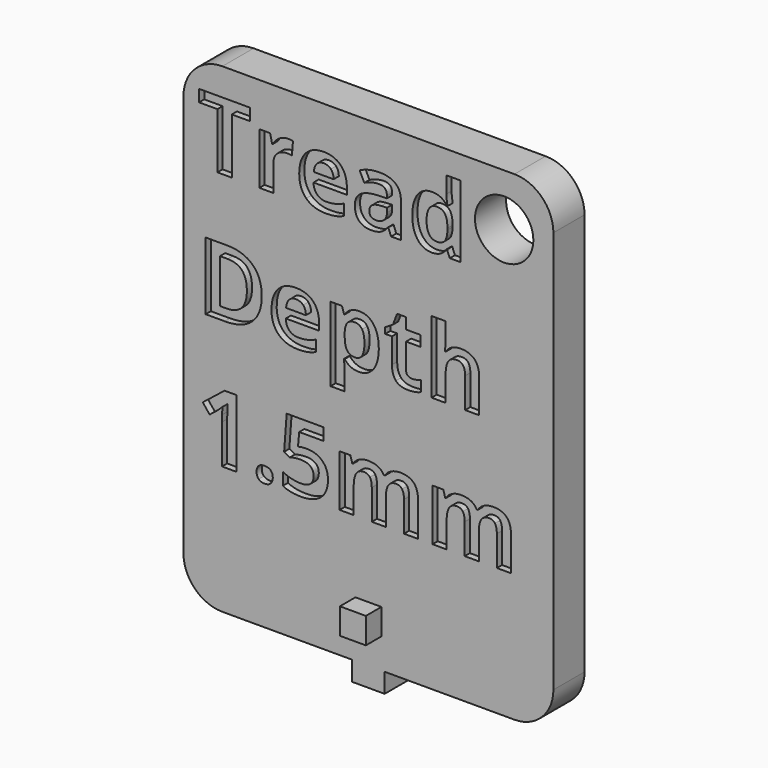
from build123d import *

# Parameters (mm, degrees)
F0_W         = 2
F0_H         = 2
F0_R         = 2.25
F1_DEPTH     = 3
F0_TEXT_SIZE = 7.2916666667
F2_DEPTH     = 2.5
F3_DEPTH     = 4.5
F4_R         = 3


# Not quite as in the source:
# - Text() gives the source's letters only with a copy of the font that has no kerning and outlines rounded to 1/6400 em; it was checked with that copy


with BuildPart() as f1:
    # F0 (on Front) → F1 (new body)
    with BuildSketch(Plane.XZ):
        Polygon((-22.369877694, 72.3569517974), (-50.869877694, 72.3569517974), (-50.869877694, 35.3569517974), (-37.869877694, 35.3569517974), (-37.869877694, 33.8569517974), (-35.369877694, 33.8569517974), (-35.369877694, 35.3569517974), (-22.369877694, 35.3569517974), align=None)
        with BuildLine():
            Line((-46.8008372088, 50.4102206628), (-46.8008372088, 45.2046542565))
            Line((-46.8008372088, 45.2046542565), (-47.9014231463, 45.2046542565))
            Line((-47.9014231463, 45.2046542565), (-47.9014231463, 48.2170240482))
            Line((-47.9014231463, 48.2170240482), (-47.8900299172, 48.711490194))
            Line((-47.8900299172, 48.711490194), (-47.8729400734, 49.2526685794))
            add(Edge.make_bspline(
                [(-47.8729400734, 49.2526685794), (-48.1463775734, 48.9792310794), (-48.2534739276, 48.8937818607)],
                knots=[0, 0, 0, 1, 1, 1], degree=2))
            Line((-48.2534739276, 48.8937818607), (-48.8516184588, 48.4129875898))
            Line((-48.8516184588, 48.4129875898), (-49.382542938, 49.0749342044))
            Line((-49.382542938, 49.0749342044), (-47.7054596047, 50.4102206628))
            Line((-47.7054596047, 50.4102206628), (-46.8008372088, 50.4102206628))
        make_face(mode=Mode.SUBTRACT)
        with BuildLine():
            add(Edge.make_bspline(
                [(-45.0707753599, 45.2673170169), (-45.2342681984, 45.4256829023), (-45.2342681984, 45.7139316003)],
                knots=[0, 0, 0, 1, 1, 1], degree=2))
            add(Edge.make_bspline(
                [(-45.2342681984, 45.7139316003), (-45.2342681984, 46.0124342044), (-45.0741933286, 46.1656731367)],
                knots=[0, 0, 0, 1, 1, 1], degree=2))
            add(Edge.make_bspline(
                [(-45.0741933286, 46.1656731367), (-44.9141184588, 46.318912069), (-44.6076405942, 46.318912069)],
                knots=[0, 0, 0, 1, 1, 1], degree=2))
            add(Edge.make_bspline(
                [(-44.6076405942, 46.318912069), (-44.3125559588, 46.318912069), (-44.1507721047, 46.162255168)],
                knots=[0, 0, 0, 1, 1, 1], degree=2))
            add(Edge.make_bspline(
                [(-44.1507721047, 46.162255168), (-43.9889882505, 46.0055982669), (-43.9889882505, 45.7139316003)],
                knots=[0, 0, 0, 1, 1, 1], degree=2))
            add(Edge.make_bspline(
                [(-43.9889882505, 45.7139316003), (-43.9889882505, 45.4325188398), (-44.152481089, 45.2707349857)],
                knots=[0, 0, 0, 1, 1, 1], degree=2))
            add(Edge.make_bspline(
                [(-44.152481089, 45.2707349857), (-44.3159739276, 45.1089511315), (-44.6076405942, 45.1089511315)],
                knots=[0, 0, 0, 1, 1, 1], degree=2))
            add(Edge.make_bspline(
                [(-44.6076405942, 45.1089511315), (-44.9072825213, 45.1089511315), (-45.0707753599, 45.2673170169)],
                knots=[0, 0, 0, 1, 1, 1], degree=2))
        make_face(mode=Mode.SUBTRACT)
        with BuildLine():
            add(Edge.make_bspline(
                [(-41.9233958026, 48.4802076419), (-41.7057851255, 48.5303378503), (-41.3856353859, 48.5303378503)],
                knots=[0, 0, 0, 1, 1, 1], degree=2))
            add(Edge.make_bspline(
                [(-41.3856353859, 48.5303378503), (-40.6314036151, 48.5303378503), (-40.1842193703, 48.1065097253)],
                knots=[0, 0, 0, 1, 1, 1], degree=2))
            add(Edge.make_bspline(
                [(-40.1842193703, 48.1065097253), (-39.7370351255, 47.6826816003), (-39.7370351255, 46.9455396732)],
                knots=[0, 0, 0, 1, 1, 1], degree=2))
            add(Edge.make_bspline(
                [(-39.7370351255, 46.9455396732), (-39.7370351255, 46.0739576419), (-40.2747955422, 45.6034172773)],
                knots=[0, 0, 0, 1, 1, 1], degree=2))
            add(Edge.make_bspline(
                [(-40.2747955422, 45.6034172773), (-40.8125559588, 45.1328769128), (-41.8128814797, 45.1328769128)],
                knots=[0, 0, 0, 1, 1, 1], degree=2))
            add(Edge.make_bspline(
                [(-41.8128814797, 45.1328769128), (-42.6821848651, 45.1328769128), (-43.2153879901, 45.4142896732)],
                knots=[0, 0, 0, 1, 1, 1], degree=2))
            Line((-43.2153879901, 45.4142896732), (-43.2153879901, 46.3656243086))
            add(Edge.make_bspline(
                [(-43.2153879901, 46.3656243086), (-42.9351145526, 46.2163730065), (-42.5608469745, 46.1218092044)],
                knots=[0, 0, 0, 1, 1, 1], degree=2))
            add(Edge.make_bspline(
                [(-42.5608469745, 46.1218092044), (-42.1865793963, 46.0272454023), (-41.8527577817, 46.0272454023)],
                knots=[0, 0, 0, 1, 1, 1], degree=2))
            add(Edge.make_bspline(
                [(-41.8527577817, 46.0272454023), (-40.8444570005, 46.0272454023), (-40.8444570005, 46.8532545169)],
                knots=[0, 0, 0, 1, 1, 1], degree=2))
            add(Edge.make_bspline(
                [(-40.8444570005, 46.8532545169), (-40.8444570005, 47.6405266523), (-41.8880767922, 47.6405266523)],
                knots=[0, 0, 0, 1, 1, 1], degree=2))
            add(Edge.make_bspline(
                [(-41.8880767922, 47.6405266523), (-42.0760650734, 47.6405266523), (-42.3039296567, 47.6029289961)],
                knots=[0, 0, 0, 1, 1, 1], degree=2))
            add(Edge.make_bspline(
                [(-42.3039296567, 47.6029289961), (-42.5317942401, 47.5653313398), (-42.6742096047, 47.522037069)],
                knots=[0, 0, 0, 1, 1, 1], degree=2))
            Line((-42.6742096047, 47.522037069), (-43.1128489276, 47.7578769128))
            Line((-43.1128489276, 47.7578769128), (-42.9168853859, 50.4102206628))
            Line((-42.9168853859, 50.4102206628), (-40.0936431984, 50.4102206628))
            Line((-40.0936431984, 50.4102206628), (-40.0936431984, 49.477115194))
            Line((-40.0936431984, 49.477115194), (-41.9518788755, 49.477115194))
            Line((-41.9518788755, 49.477115194), (-42.0475820005, 48.4551425378))
            Line((-42.0475820005, 48.4551425378), (-41.9233958026, 48.4802076419))
        make_face(mode=Mode.SUBTRACT)
        with Locations((-36.619877694, 38.6735366881)):
            Rectangle(F0_W, F0_H, mode=Mode.SUBTRACT)
        with BuildLine():
            Line((-35.2765859067, 47.2018873294), (-35.2765859067, 45.2046542565))
            Line((-35.2765859067, 45.2046542565), (-36.3623606463, 45.2046542565))
            Line((-36.3623606463, 45.2046542565), (-36.3623606463, 47.5300123294))
            add(Edge.make_bspline(
                [(-36.3623606463, 47.5300123294), (-36.3623606463, 47.9606763919), (-36.5064849953, 48.1760084232)],
                knots=[0, 0, 0, 1, 1, 1], degree=2))
            add(Edge.make_bspline(
                [(-36.5064849953, 48.1760084232), (-36.6506093442, 48.3913404544), (-36.9605051776, 48.3913404544)],
                knots=[0, 0, 0, 1, 1, 1], degree=2))
            add(Edge.make_bspline(
                [(-36.9605051776, 48.3913404544), (-37.3774973651, 48.3913404544), (-37.5660553078, 48.0848625898)],
                knots=[0, 0, 0, 1, 1, 1], degree=2))
            add(Edge.make_bspline(
                [(-37.5660553078, 48.0848625898), (-37.7546132505, 47.7783847253), (-37.7546132505, 47.0777011315)],
                knots=[0, 0, 0, 1, 1, 1], degree=2))
            Line((-37.7546132505, 47.0777011315), (-37.7546132505, 45.2046542565))
            Line((-37.7546132505, 45.2046542565), (-38.8403879901, 45.2046542565))
            Line((-38.8403879901, 45.2046542565), (-38.8403879901, 49.1854485273))
            Line((-38.8403879901, 49.1854485273), (-38.0109609067, 49.1854485273))
            Line((-38.0109609067, 49.1854485273), (-37.8651275734, 48.6761711836))
            Line((-37.8651275734, 48.6761711836), (-37.8047434588, 48.6761711836))
            add(Edge.make_bspline(
                [(-37.8047434588, 48.6761711836), (-37.6440989276, 48.9507480065), (-37.3416086932, 49.1051262617)],
                knots=[0, 0, 0, 1, 1, 1], degree=2))
            add(Edge.make_bspline(
                [(-37.3416086932, 49.1051262617), (-37.0391184588, 49.2595045169), (-36.6471913755, 49.2595045169)],
                knots=[0, 0, 0, 1, 1, 1], degree=2))
            add(Edge.make_bspline(
                [(-36.6471913755, 49.2595045169), (-35.7539622088, 49.2595045169), (-35.4360911151, 48.6761711836)],
                knots=[0, 0, 0, 1, 1, 1], degree=2))
            Line((-35.4360911151, 48.6761711836), (-35.3403879901, 48.6761711836))
            add(Edge.make_bspline(
                [(-35.3403879901, 48.6761711836), (-35.1797434588, 48.9541659753), (-34.8687083026, 49.1068352461)],
                knots=[0, 0, 0, 1, 1, 1], degree=2))
            add(Edge.make_bspline(
                [(-34.8687083026, 49.1068352461), (-34.5576731463, 49.2595045169), (-34.165746063, 49.2595045169)],
                knots=[0, 0, 0, 1, 1, 1], degree=2))
            add(Edge.make_bspline(
                [(-34.165746063, 49.2595045169), (-33.4889882505, 49.2595045169), (-33.1420644224, 48.9125806888)],
                knots=[0, 0, 0, 1, 1, 1], degree=2))
            add(Edge.make_bspline(
                [(-33.1420644224, 48.9125806888), (-32.7951405942, 48.5656568607), (-32.7951405942, 47.8000318607)],
                knots=[0, 0, 0, 1, 1, 1], degree=2))
            Line((-32.7951405942, 47.8000318607), (-32.7951405942, 45.2046542565))
            Line((-32.7951405942, 45.2046542565), (-33.8843333026, 45.2046542565))
            Line((-33.8843333026, 45.2046542565), (-33.8843333026, 47.5300123294))
            add(Edge.make_bspline(
                [(-33.8843333026, 47.5300123294), (-33.8843333026, 47.9606763919), (-34.0284576515, 48.1760084232)],
                knots=[0, 0, 0, 1, 1, 1], degree=2))
            add(Edge.make_bspline(
                [(-34.0284576515, 48.1760084232), (-34.1725820005, 48.3913404544), (-34.4824778338, 48.3913404544)],
                knots=[0, 0, 0, 1, 1, 1], degree=2))
            add(Edge.make_bspline(
                [(-34.4824778338, 48.3913404544), (-34.8812408547, 48.3913404544), (-35.0789133807, 48.1065097253)],
                knots=[0, 0, 0, 1, 1, 1], degree=2))
            add(Edge.make_bspline(
                [(-35.0789133807, 48.1065097253), (-35.2765859067, 47.8216789961), (-35.2765859067, 47.2018873294)],
                knots=[0, 0, 0, 1, 1, 1], degree=2))
        make_face(mode=Mode.SUBTRACT)
        with BuildLine():
            Line((-28.1170806984, 47.2018873294), (-28.1170806984, 45.2046542565))
            Line((-28.1170806984, 45.2046542565), (-29.202855438, 45.2046542565))
            Line((-29.202855438, 45.2046542565), (-29.202855438, 47.5300123294))
            add(Edge.make_bspline(
                [(-29.202855438, 47.5300123294), (-29.202855438, 47.9606763919), (-29.346979787, 48.1760084232)],
                knots=[0, 0, 0, 1, 1, 1], degree=2))
            add(Edge.make_bspline(
                [(-29.346979787, 48.1760084232), (-29.4911041359, 48.3913404544), (-29.8009999692, 48.3913404544)],
                knots=[0, 0, 0, 1, 1, 1], degree=2))
            add(Edge.make_bspline(
                [(-29.8009999692, 48.3913404544), (-30.2179921567, 48.3913404544), (-30.4065500995, 48.0848625898)],
                knots=[0, 0, 0, 1, 1, 1], degree=2))
            add(Edge.make_bspline(
                [(-30.4065500995, 48.0848625898), (-30.5951080422, 47.7783847253), (-30.5951080422, 47.0777011315)],
                knots=[0, 0, 0, 1, 1, 1], degree=2))
            Line((-30.5951080422, 47.0777011315), (-30.5951080422, 45.2046542565))
            Line((-30.5951080422, 45.2046542565), (-31.6808827817, 45.2046542565))
            Line((-31.6808827817, 45.2046542565), (-31.6808827817, 49.1854485273))
            Line((-31.6808827817, 49.1854485273), (-30.8514556984, 49.1854485273))
            Line((-30.8514556984, 49.1854485273), (-30.7056223651, 48.6761711836))
            Line((-30.7056223651, 48.6761711836), (-30.6452382505, 48.6761711836))
            add(Edge.make_bspline(
                [(-30.6452382505, 48.6761711836), (-30.4845937192, 48.9507480065), (-30.1821034849, 49.1051262617)],
                knots=[0, 0, 0, 1, 1, 1], degree=2))
            add(Edge.make_bspline(
                [(-30.1821034849, 49.1051262617), (-29.8796132505, 49.2595045169), (-29.4876861672, 49.2595045169)],
                knots=[0, 0, 0, 1, 1, 1], degree=2))
            add(Edge.make_bspline(
                [(-29.4876861672, 49.2595045169), (-28.5944570005, 49.2595045169), (-28.2765859067, 48.6761711836)],
                knots=[0, 0, 0, 1, 1, 1], degree=2))
            Line((-28.2765859067, 48.6761711836), (-28.1808827817, 48.6761711836))
            add(Edge.make_bspline(
                [(-28.1808827817, 48.6761711836), (-28.0202382505, 48.9541659753), (-27.7092030942, 49.1068352461)],
                knots=[0, 0, 0, 1, 1, 1], degree=2))
            add(Edge.make_bspline(
                [(-27.7092030942, 49.1068352461), (-27.398167938, 49.2595045169), (-27.0062408547, 49.2595045169)],
                knots=[0, 0, 0, 1, 1, 1], degree=2))
            add(Edge.make_bspline(
                [(-27.0062408547, 49.2595045169), (-26.3294830422, 49.2595045169), (-25.982559214, 48.9125806888)],
                knots=[0, 0, 0, 1, 1, 1], degree=2))
            add(Edge.make_bspline(
                [(-25.982559214, 48.9125806888), (-25.6356353859, 48.5656568607), (-25.6356353859, 47.8000318607)],
                knots=[0, 0, 0, 1, 1, 1], degree=2))
            Line((-25.6356353859, 47.8000318607), (-25.6356353859, 45.2046542565))
            Line((-25.6356353859, 45.2046542565), (-26.7248280942, 45.2046542565))
            Line((-26.7248280942, 45.2046542565), (-26.7248280942, 47.5300123294))
            add(Edge.make_bspline(
                [(-26.7248280942, 47.5300123294), (-26.7248280942, 47.9606763919), (-26.8689524432, 48.1760084232)],
                knots=[0, 0, 0, 1, 1, 1], degree=2))
            add(Edge.make_bspline(
                [(-26.8689524432, 48.1760084232), (-27.0130767922, 48.3913404544), (-27.3229726255, 48.3913404544)],
                knots=[0, 0, 0, 1, 1, 1], degree=2))
            add(Edge.make_bspline(
                [(-27.3229726255, 48.3913404544), (-27.7217356463, 48.3913404544), (-27.9194081724, 48.1065097253)],
                knots=[0, 0, 0, 1, 1, 1], degree=2))
            add(Edge.make_bspline(
                [(-27.9194081724, 48.1065097253), (-28.1170806984, 47.8216789961), (-28.1170806984, 47.2018873294)],
                knots=[0, 0, 0, 1, 1, 1], degree=2))
        make_face(mode=Mode.SUBTRACT)
        with BuildLine():
            add(Edge.make_bspline(
                [(-45.5441640317, 59.6541171471), (-44.8389231463, 58.9813469648), (-44.8389231463, 57.7736646732)],
                knots=[0, 0, 0, 1, 1, 1], degree=2))
            add(Edge.make_bspline(
                [(-44.8389231463, 57.7736646732), (-44.8389231463, 56.4885084232), (-45.5709381203, 55.8049146732)],
                knots=[0, 0, 0, 1, 1, 1], degree=2))
            add(Edge.make_bspline(
                [(-45.5709381203, 55.8049146732), (-46.3029530942, 55.1213209232), (-47.6838124692, 55.1213209232)],
                knots=[0, 0, 0, 1, 1, 1], degree=2))
            Line((-47.6838124692, 55.1213209232), (-49.1580963234, 55.1213209232))
            Line((-49.1580963234, 55.1213209232), (-49.1580963234, 60.3268873294))
            Line((-49.1580963234, 60.3268873294), (-47.5243072609, 60.3268873294))
            add(Edge.make_bspline(
                [(-47.5243072609, 60.3268873294), (-46.2494049172, 60.3268873294), (-45.5441640317, 59.6541171471)],
                knots=[0, 0, 0, 1, 1, 1], degree=2))
        make_face(mode=Mode.SUBTRACT)
        with BuildLine():
            add(Edge.make_bspline(
                [(-41.2534739276, 55.1190422773), (-41.5770416359, 55.0495435794), (-42.0441640317, 55.0495435794)],
                knots=[0, 0, 0, 1, 1, 1], degree=2))
            add(Edge.make_bspline(
                [(-42.0441640317, 55.0495435794), (-43.0046132505, 55.0495435794), (-43.5457916359, 55.5804680586)],
                knots=[0, 0, 0, 1, 1, 1], degree=2))
            add(Edge.make_bspline(
                [(-43.5457916359, 55.5804680586), (-44.0869700213, 56.1113925378), (-44.0869700213, 57.0832349857)],
                knots=[0, 0, 0, 1, 1, 1], degree=2))
            add(Edge.make_bspline(
                [(-44.0869700213, 57.0832349857), (-44.0869700213, 58.0835605065), (-43.5868072609, 58.629865845)],
                knots=[0, 0, 0, 1, 1, 1], degree=2))
            add(Edge.make_bspline(
                [(-43.5868072609, 58.629865845), (-43.0866445005, 59.1761711836), (-42.2036692401, 59.1761711836)],
                knots=[0, 0, 0, 1, 1, 1], degree=2))
            add(Edge.make_bspline(
                [(-42.2036692401, 59.1761711836), (-41.3605702817, 59.1761711836), (-40.8905995786, 58.6959465742)],
                knots=[0, 0, 0, 1, 1, 1], degree=2))
            add(Edge.make_bspline(
                [(-40.8905995786, 58.6959465742), (-40.4206288755, 58.2157219648), (-40.4206288755, 57.3680657148)],
                knots=[0, 0, 0, 1, 1, 1], degree=2))
            Line((-40.4206288755, 57.3680657148), (-40.4206288755, 56.8405592044))
            Line((-40.4206288755, 56.8405592044), (-42.9875234067, 56.8405592044))
            add(Edge.make_bspline(
                [(-42.9875234067, 56.8405592044), (-42.9692942401, 56.3779941003), (-42.7129465838, 56.1182284753)],
                knots=[0, 0, 0, 1, 1, 1], degree=2))
            add(Edge.make_bspline(
                [(-42.7129465838, 56.1182284753), (-42.4565989276, 55.8584628503), (-41.9940338234, 55.8584628503)],
                knots=[0, 0, 0, 1, 1, 1], degree=2))
            add(Edge.make_bspline(
                [(-41.9940338234, 55.8584628503), (-41.6340077817, 55.8584628503), (-41.3138580422, 55.9330885013)],
                knots=[0, 0, 0, 1, 1, 1], degree=2))
            add(Edge.make_bspline(
                [(-41.3138580422, 55.9330885013), (-40.9937083026, 56.0077141523), (-40.6450754901, 56.1717766523)],
                knots=[0, 0, 0, 1, 1, 1], degree=2))
            Line((-40.6450754901, 56.1717766523), (-40.6450754901, 55.3309563398))
            add(Edge.make_bspline(
                [(-40.6450754901, 55.3309563398), (-40.9299062192, 55.1885409753), (-41.2534739276, 55.1190422773)],
                knots=[0, 0, 0, 1, 1, 1], degree=2))
        make_face(mode=Mode.SUBTRACT)
        with BuildLine():
            add(Edge.make_bspline(
                [(-36.5400950213, 55.2956373294), (-36.8853098651, 55.0495435794), (-37.351292938, 55.0495435794)],
                knots=[0, 0, 0, 1, 1, 1], degree=2))
            add(Edge.make_bspline(
                [(-37.351292938, 55.0495435794), (-38.0531158547, 55.0495435794), (-38.4518788755, 55.5588209232)],
                knots=[0, 0, 0, 1, 1, 1], degree=2))
            Line((-38.4518788755, 55.5588209232), (-38.5088450213, 55.5588209232))
            add(Edge.make_bspline(
                [(-38.5088450213, 55.5588209232), (-38.4518788755, 55.0609368086), (-38.4518788755, 54.9823235273)],
                knots=[0, 0, 0, 1, 1, 1], degree=2))
            Line((-38.4518788755, 54.9823235273), (-38.4518788755, 53.3690422773))
            Line((-38.4518788755, 53.3690422773), (-39.5376536151, 53.3690422773))
            Line((-39.5376536151, 53.3690422773), (-39.5376536151, 59.102115194))
            Line((-39.5376536151, 59.102115194), (-38.6546783547, 59.102115194))
            Line((-38.6546783547, 59.102115194), (-38.5020090838, 58.5860019128))
            Line((-38.5020090838, 58.5860019128), (-38.4518788755, 58.5860019128))
            add(Edge.make_bspline(
                [(-38.4518788755, 58.5860019128), (-38.0702056984, 59.1761711836), (-37.3228098651, 59.1761711836)],
                knots=[0, 0, 0, 1, 1, 1], degree=2))
            add(Edge.make_bspline(
                [(-37.3228098651, 59.1761711836), (-36.6175689797, 59.1761711836), (-36.2188059588, 58.6315748294)],
                knots=[0, 0, 0, 1, 1, 1], degree=2))
            add(Edge.make_bspline(
                [(-36.2188059588, 58.6315748294), (-35.820042938, 58.0869784753), (-35.820042938, 57.1185539961)],
                knots=[0, 0, 0, 1, 1, 1], degree=2))
            add(Edge.make_bspline(
                [(-35.820042938, 57.1185539961), (-35.820042938, 56.4816724857), (-36.0074615578, 56.0117017825)],
                knots=[0, 0, 0, 1, 1, 1], degree=2))
            add(Edge.make_bspline(
                [(-36.0074615578, 56.0117017825), (-36.1948801776, 55.5417310794), (-36.5400950213, 55.2956373294)],
                knots=[0, 0, 0, 1, 1, 1], degree=2))
        make_face(mode=Mode.SUBTRACT)
        Polygon((-47.1494700213, 69.3252597253), (-47.1494700213, 65.0379875898), (-48.2534739276, 65.0379875898), (-48.2534739276, 69.3252597253), (-49.6673736672, 69.3252597253), (-49.6673736672, 70.2435539961), (-45.7367096047, 70.2435539961), (-45.7367096047, 69.3252597253), align=None, mode=Mode.SUBTRACT)
        with BuildLine():
            add(Edge.make_bspline(
                [(-43.4848378599, 68.8883293867), (-43.1698150734, 69.0928378503), (-42.7995351255, 69.0928378503)],
                knots=[0, 0, 0, 1, 1, 1], degree=2))
            add(Edge.make_bspline(
                [(-42.7995351255, 69.0928378503), (-42.5785064797, 69.0928378503), (-42.4326731463, 69.0609368086)],
                knots=[0, 0, 0, 1, 1, 1], degree=2))
            Line((-42.4326731463, 69.0609368086), (-42.5147043963, 68.043521444))
            add(Edge.make_bspline(
                [(-42.5147043963, 68.043521444), (-42.6468658547, 68.0788404544), (-42.8348541359, 68.0788404544)],
                knots=[0, 0, 0, 1, 1, 1], degree=2))
            add(Edge.make_bspline(
                [(-42.8348541359, 68.0788404544), (-43.3543853859, 68.0788404544), (-43.6449127297, 67.8116692305)],
                knots=[0, 0, 0, 1, 1, 1], degree=2))
            add(Edge.make_bspline(
                [(-43.6449127297, 67.8116692305), (-43.9354400734, 67.5444980065), (-43.9354400734, 67.0637037357)],
                knots=[0, 0, 0, 1, 1, 1], degree=2))
            Line((-43.9354400734, 67.0637037357), (-43.9354400734, 65.0379875898))
            Line((-43.9354400734, 65.0379875898), (-45.021214813, 65.0379875898))
            Line((-45.021214813, 65.0379875898), (-45.021214813, 69.0187818607))
            Line((-45.021214813, 69.0187818607), (-44.1986236672, 69.0187818607))
            Line((-44.1986236672, 69.0187818607), (-44.0379791359, 68.3488599857))
            Line((-44.0379791359, 68.3488599857), (-43.9855702817, 68.3488599857))
            add(Edge.make_bspline(
                [(-43.9855702817, 68.3488599857), (-43.7998606463, 68.6838209232), (-43.4848378599, 68.8883293867)],
                knots=[0, 0, 0, 1, 1, 1], degree=2))
        make_face(mode=Mode.SUBTRACT)
        with BuildLine():
            add(Edge.make_bspline(
                [(-39.1183827817, 65.035708944), (-39.4419504901, 64.9662102461), (-39.9090728859, 64.9662102461)],
                knots=[0, 0, 0, 1, 1, 1], degree=2))
            add(Edge.make_bspline(
                [(-39.9090728859, 64.9662102461), (-40.8695221047, 64.9662102461), (-41.4107004901, 65.4971347253)],
                knots=[0, 0, 0, 1, 1, 1], degree=2))
            add(Edge.make_bspline(
                [(-41.4107004901, 65.4971347253), (-41.9518788755, 66.0280592044), (-41.9518788755, 66.9999016523)],
                knots=[0, 0, 0, 1, 1, 1], degree=2))
            add(Edge.make_bspline(
                [(-41.9518788755, 66.9999016523), (-41.9518788755, 68.0002271732), (-41.4517161151, 68.5465325117)],
                knots=[0, 0, 0, 1, 1, 1], degree=2))
            add(Edge.make_bspline(
                [(-41.4517161151, 68.5465325117), (-40.9515533547, 69.0928378503), (-40.0685780942, 69.0928378503)],
                knots=[0, 0, 0, 1, 1, 1], degree=2))
            add(Edge.make_bspline(
                [(-40.0685780942, 69.0928378503), (-39.2254791359, 69.0928378503), (-38.7555084328, 68.6126132409)],
                knots=[0, 0, 0, 1, 1, 1], degree=2))
            add(Edge.make_bspline(
                [(-38.7555084328, 68.6126132409), (-38.2855377297, 68.1323886315), (-38.2855377297, 67.2847323815)],
                knots=[0, 0, 0, 1, 1, 1], degree=2))
            Line((-38.2855377297, 67.2847323815), (-38.2855377297, 66.7572258711))
            Line((-38.2855377297, 66.7572258711), (-40.8524322609, 66.7572258711))
            add(Edge.make_bspline(
                [(-40.8524322609, 66.7572258711), (-40.8342030942, 66.2946607669), (-40.577855438, 66.0348951419)],
                knots=[0, 0, 0, 1, 1, 1], degree=2))
            add(Edge.make_bspline(
                [(-40.577855438, 66.0348951419), (-40.3215077817, 65.7751295169), (-39.8589426776, 65.7751295169)],
                knots=[0, 0, 0, 1, 1, 1], degree=2))
            add(Edge.make_bspline(
                [(-39.8589426776, 65.7751295169), (-39.4989166359, 65.7751295169), (-39.1787668963, 65.849755168)],
                knots=[0, 0, 0, 1, 1, 1], degree=2))
            add(Edge.make_bspline(
                [(-39.1787668963, 65.849755168), (-38.8586171567, 65.924380819), (-38.5099843442, 66.088443319)],
                knots=[0, 0, 0, 1, 1, 1], degree=2))
            Line((-38.5099843442, 66.088443319), (-38.5099843442, 65.2476230065))
            add(Edge.make_bspline(
                [(-38.5099843442, 65.2476230065), (-38.7948150734, 65.1052076419), (-39.1183827817, 65.035708944)],
                knots=[0, 0, 0, 1, 1, 1], degree=2))
        make_face(mode=Mode.SUBTRACT)
        with BuildLine():
            add(Edge.make_bspline(
                [(-33.5903879901, 56.025943319), (-33.4605051776, 55.9154289961), (-33.2463124692, 55.9154289961)],
                knots=[0, 0, 0, 1, 1, 1], degree=2))
            add(Edge.make_bspline(
                [(-33.2463124692, 55.9154289961), (-32.9614817401, 55.9154289961), (-32.5627187192, 56.039615194)],
                knots=[0, 0, 0, 1, 1, 1], degree=2))
            Line((-32.5627187192, 56.039615194), (-32.5627187192, 55.2318352461))
            add(Edge.make_bspline(
                [(-32.5627187192, 55.2318352461), (-32.9683176776, 55.0495435794), (-33.5596262713, 55.0495435794)],
                knots=[0, 0, 0, 1, 1, 1], degree=2))
            add(Edge.make_bspline(
                [(-33.5596262713, 55.0495435794), (-34.2113189797, 55.0495435794), (-34.5086822609, 55.3793775638)],
                knots=[0, 0, 0, 1, 1, 1], degree=2))
            add(Edge.make_bspline(
                [(-34.5086822609, 55.3793775638), (-34.8060455422, 55.7092115482), (-34.8060455422, 56.367740194)],
                knots=[0, 0, 0, 1, 1, 1], degree=2))
            Line((-34.8060455422, 56.367740194), (-34.8060455422, 58.2863599857))
            Line((-34.8060455422, 58.2863599857), (-35.3255767922, 58.2863599857))
            Line((-35.3255767922, 58.2863599857), (-35.3255767922, 58.7455071211))
            Line((-35.3255767922, 58.7455071211), (-34.7274322609, 59.1089511315))
            Line((-34.7274322609, 59.1089511315), (-34.4141184588, 59.949771444))
            Line((-34.4141184588, 59.949771444), (-33.7202708026, 59.949771444))
            Line((-33.7202708026, 59.949771444), (-33.7202708026, 59.102115194))
            Line((-33.7202708026, 59.102115194), (-32.6060129901, 59.102115194))
            Line((-32.6060129901, 59.102115194), (-32.6060129901, 58.2863599857))
            Line((-32.6060129901, 58.2863599857), (-33.7202708026, 58.2863599857))
            Line((-33.7202708026, 58.2863599857), (-33.7202708026, 56.367740194))
            add(Edge.make_bspline(
                [(-33.7202708026, 56.367740194), (-33.7202708026, 56.1364576419), (-33.5903879901, 56.025943319)],
                knots=[0, 0, 0, 1, 1, 1], degree=2))
        make_face(mode=Mode.SUBTRACT)
        with BuildLine():
            Line((-28.0840403338, 57.7166985273), (-28.0840403338, 55.1213209232))
            Line((-28.0840403338, 55.1213209232), (-29.1698150734, 55.1213209232))
            Line((-29.1698150734, 55.1213209232), (-29.1698150734, 57.4466789961))
            add(Edge.make_bspline(
                [(-29.1698150734, 57.4466789961), (-29.1698150734, 58.3080071211), (-29.8112538755, 58.3080071211)],
                knots=[0, 0, 0, 1, 1, 1], degree=2))
            add(Edge.make_bspline(
                [(-29.8112538755, 58.3080071211), (-30.2669830422, 58.3080071211), (-30.4697825213, 57.9981112878)],
                knots=[0, 0, 0, 1, 1, 1], degree=2))
            add(Edge.make_bspline(
                [(-30.4697825213, 57.9981112878), (-30.6725820005, 57.6882154544), (-30.6725820005, 56.9943677982)],
                knots=[0, 0, 0, 1, 1, 1], degree=2))
            Line((-30.6725820005, 56.9943677982), (-30.6725820005, 55.1213209232))
            Line((-30.6725820005, 55.1213209232), (-31.7583567401, 55.1213209232))
            Line((-31.7583567401, 55.1213209232), (-31.7583567401, 60.6618482669))
            Line((-31.7583567401, 60.6618482669), (-30.6725820005, 60.6618482669))
            Line((-30.6725820005, 60.6618482669), (-30.6725820005, 59.5327792565))
            add(Edge.make_bspline(
                [(-30.6725820005, 59.5327792565), (-30.6725820005, 59.4006177982), (-30.6976471047, 58.9129875898)],
                knots=[0, 0, 0, 1, 1, 1], degree=2))
            Line((-30.6976471047, 58.9129875898), (-30.7227122088, 58.5928378503))
            Line((-30.7227122088, 58.5928378503), (-30.665746063, 58.5928378503))
            add(Edge.make_bspline(
                [(-30.665746063, 58.5928378503), (-30.3023020526, 59.1761711836), (-29.5116119484, 59.1761711836)],
                knots=[0, 0, 0, 1, 1, 1], degree=2))
            add(Edge.make_bspline(
                [(-29.5116119484, 59.1761711836), (-28.8097890317, 59.1761711836), (-28.4469146828, 58.7990552982)],
                knots=[0, 0, 0, 1, 1, 1], degree=2))
            add(Edge.make_bspline(
                [(-28.4469146828, 58.7990552982), (-28.0840403338, 58.4219394128), (-28.0840403338, 57.7166985273)],
                knots=[0, 0, 0, 1, 1, 1], degree=2))
        make_face(mode=Mode.SUBTRACT)
        with BuildLine():
            Line((-34.1167551776, 65.0379875898), (-34.8744049172, 65.0379875898))
            Line((-34.8744049172, 65.0379875898), (-35.0851796567, 65.5791659753))
            Line((-35.0851796567, 65.5791659753), (-35.1136627297, 65.5791659753))
            add(Edge.make_bspline(
                [(-35.1136627297, 65.5791659753), (-35.3871002297, 65.2339511315), (-35.6776275734, 65.1000806888)],
                knots=[0, 0, 0, 1, 1, 1], degree=2))
            add(Edge.make_bspline(
                [(-35.6776275734, 65.1000806888), (-35.9681549172, 64.9662102461), (-36.4341379901, 64.9662102461)],
                knots=[0, 0, 0, 1, 1, 1], degree=2))
            add(Edge.make_bspline(
                [(-36.4341379901, 64.9662102461), (-37.0072174172, 64.9662102461), (-37.3364817401, 65.2943352461)],
                knots=[0, 0, 0, 1, 1, 1], degree=2))
            add(Edge.make_bspline(
                [(-37.3364817401, 65.2943352461), (-37.665746063, 65.6224602461), (-37.665746063, 66.2274407148)],
                knots=[0, 0, 0, 1, 1, 1], degree=2))
            add(Edge.make_bspline(
                [(-37.665746063, 66.2274407148), (-37.665746063, 66.8609042565), (-37.2225494484, 67.1616855065)],
                knots=[0, 0, 0, 1, 1, 1], degree=2))
            add(Edge.make_bspline(
                [(-37.2225494484, 67.1616855065), (-36.7793528338, 67.4624667565), (-35.8861236672, 67.4943677982)],
                knots=[0, 0, 0, 1, 1, 1], degree=2))
            Line((-35.8861236672, 67.4943677982), (-35.1945546567, 67.5160149336))
            Line((-35.1945546567, 67.5160149336), (-35.1945546567, 67.6903313398))
            add(Edge.make_bspline(
                [(-35.1945546567, 67.6903313398), (-35.1945546567, 68.2953118086), (-35.8143463234, 68.2953118086)],
                knots=[0, 0, 0, 1, 1, 1], degree=2))
            add(Edge.make_bspline(
                [(-35.8143463234, 68.2953118086), (-36.2917226255, 68.2953118086), (-36.9365793963, 68.0070631107)],
                knots=[0, 0, 0, 1, 1, 1], degree=2))
            Line((-36.9365793963, 68.0070631107), (-37.2954661151, 68.740787069))
            add(Edge.make_bspline(
                [(-37.2954661151, 68.740787069), (-36.6084543963, 69.1008131107), (-35.7721913755, 69.1008131107)],
                knots=[0, 0, 0, 1, 1, 1], degree=2))
            add(Edge.make_bspline(
                [(-35.7721913755, 69.1008131107), (-34.9712473651, 69.1008131107), (-34.5440012713, 68.7516106367)],
                knots=[0, 0, 0, 1, 1, 1], degree=2))
            add(Edge.make_bspline(
                [(-34.5440012713, 68.7516106367), (-34.1167551776, 68.4024081628), (-34.1167551776, 67.6903313398)],
                knots=[0, 0, 0, 1, 1, 1], degree=2))
            Line((-34.1167551776, 67.6903313398), (-34.1167551776, 65.0379875898))
        make_face(mode=Mode.SUBTRACT)
        with BuildLine():
            add(Edge.make_bspline(
                [(-30.6087799172, 65.5541008711), (-30.9790598651, 64.9662102461), (-31.7378489276, 64.9662102461)],
                knots=[0, 0, 0, 1, 1, 1], degree=2))
            add(Edge.make_bspline(
                [(-31.7378489276, 64.9662102461), (-32.4385325213, 64.9662102461), (-32.8390045265, 65.5113762617)],
                knots=[0, 0, 0, 1, 1, 1], degree=2))
            add(Edge.make_bspline(
                [(-32.8390045265, 65.5113762617), (-33.2394765317, 66.0565422773), (-33.2394765317, 67.0215487878)],
                knots=[0, 0, 0, 1, 1, 1], degree=2))
            add(Edge.make_bspline(
                [(-33.2394765317, 67.0215487878), (-33.2394765317, 68.0002271732), (-32.832168589, 68.5465325117)],
                knots=[0, 0, 0, 1, 1, 1], degree=2))
            add(Edge.make_bspline(
                [(-32.832168589, 68.5465325117), (-32.4248606463, 69.0928378503), (-31.7093658547, 69.0928378503)],
                knots=[0, 0, 0, 1, 1, 1], degree=2))
            add(Edge.make_bspline(
                [(-31.7093658547, 69.0928378503), (-30.9574127297, 69.0928378503), (-30.5620676776, 68.5095045169)],
                knots=[0, 0, 0, 1, 1, 1], degree=2))
            Line((-30.5620676776, 68.5095045169), (-30.5267486672, 68.5095045169))
            add(Edge.make_bspline(
                [(-30.5267486672, 68.5095045169), (-30.6087799172, 68.9549797773), (-30.6087799172, 69.3036125898)],
                knots=[0, 0, 0, 1, 1, 1], degree=2))
            Line((-30.6087799172, 69.3036125898), (-30.6087799172, 70.5785149336))
            Line((-30.6087799172, 70.5785149336), (-29.5195872088, 70.5785149336))
            Line((-29.5195872088, 70.5785149336), (-29.5195872088, 65.0379875898))
            Line((-29.5195872088, 65.0379875898), (-30.3524322609, 65.0379875898))
            Line((-30.3524322609, 65.0379875898), (-30.5620676776, 65.5541008711))
            Line((-30.5620676776, 65.5541008711), (-30.6087799172, 65.5541008711))
        make_face(mode=Mode.SUBTRACT)
        with Locations((-26.1633489281, 68.3512836695)):
            Circle(F0_R, mode=Mode.SUBTRACT)
    extrude(amount=F1_DEPTH)



with BuildPart() as f1b:
    # F0 (on Front) → F1, piece 2 (new body)
    with BuildSketch(Plane.XZ):
        with BuildLine():
            Line((-35.1945546567, 66.5544263919), (-35.1945546567, 66.8825513919))
            Line((-35.1945546567, 66.8825513919), (-35.614964813, 66.867740194))
            add(Edge.make_bspline(
                [(-35.614964813, 66.867740194), (-36.0889231463, 66.854068319), (-36.3202056984, 66.697411418)],
                knots=[0, 0, 0, 1, 1, 1], degree=2))
            add(Edge.make_bspline(
                [(-36.3202056984, 66.697411418), (-36.5514882505, 66.5407545169), (-36.5514882505, 66.2206047773)],
                knots=[0, 0, 0, 1, 1, 1], degree=2))
            add(Edge.make_bspline(
                [(-36.5514882505, 66.2206047773), (-36.5514882505, 65.760318319), (-36.025121063, 65.760318319)],
                knots=[0, 0, 0, 1, 1, 1], degree=2))
            add(Edge.make_bspline(
                [(-36.025121063, 65.760318319), (-35.6468658547, 65.760318319), (-35.4207102557, 65.9779289961)],
                knots=[0, 0, 0, 1, 1, 1], degree=2))
            add(Edge.make_bspline(
                [(-35.4207102557, 65.9779289961), (-35.1945546567, 66.1955396732), (-35.1945546567, 66.5544263919)],
                knots=[0, 0, 0, 1, 1, 1], degree=2))
        make_face()
    extrude(amount=F1_DEPTH)


with BuildPart() as f1c:
    # F0 (on Front) → F1, piece 3 (new body)
    with BuildSketch(Plane.XZ):
        with BuildLine():
            add(Edge.make_bspline(
                [(-41.6488189797, 58.1849602461), (-41.8516184588, 58.4037102461), (-42.1968333026, 58.4037102461)],
                knots=[0, 0, 0, 1, 1, 1], degree=2))
            add(Edge.make_bspline(
                [(-42.1968333026, 58.4037102461), (-42.5420481463, 58.4037102461), (-42.738011688, 58.1849602461)],
                knots=[0, 0, 0, 1, 1, 1], degree=2))
            add(Edge.make_bspline(
                [(-42.738011688, 58.1849602461), (-42.9339752297, 57.9662102461), (-42.9624583026, 57.5640292565)],
                knots=[0, 0, 0, 1, 1, 1], degree=2))
            Line((-42.9624583026, 57.5640292565), (-41.4380442401, 57.5640292565))
            add(Edge.make_bspline(
                [(-41.4380442401, 57.5640292565), (-41.4460195005, 57.9662102461), (-41.6488189797, 58.1849602461)],
                knots=[0, 0, 0, 1, 1, 1], degree=2))
        make_face()
    extrude(amount=F1_DEPTH)


with BuildPart() as f1d:
    # F0 (on Front) → F1, piece 4 (new body)
    with BuildSketch(Plane.XZ):
        with BuildLine():
            add(Edge.make_bspline(
                [(-47.5812734067, 56.0327792565), (-45.9862213234, 56.0327792565), (-45.9862213234, 57.7451816003)],
                knots=[0, 0, 0, 1, 1, 1], degree=2))
            add(Edge.make_bspline(
                [(-45.9862213234, 57.7451816003), (-45.9862213234, 59.4222649336), (-47.4673411151, 59.4222649336)],
                knots=[0, 0, 0, 1, 1, 1], degree=2))
            Line((-47.4673411151, 59.4222649336), (-48.0540924172, 59.4222649336))
            Line((-48.0540924172, 59.4222649336), (-48.0540924172, 56.0327792565))
            Line((-48.0540924172, 56.0327792565), (-47.5812734067, 56.0327792565))
        make_face()
    extrude(amount=F1_DEPTH)


with BuildPart() as f1e:
    # F0 (on Front) → F1, piece 5 (new body)
    with BuildSketch(Plane.XZ):
        with BuildLine():
            add(Edge.make_bspline(
                [(-37.1074778338, 58.0140618086), (-37.2874908547, 58.3080071211), (-37.6714426776, 58.3080071211)],
                knots=[0, 0, 0, 1, 1, 1], degree=2))
            add(Edge.make_bspline(
                [(-37.6714426776, 58.3080071211), (-38.0747629901, 58.3080071211), (-38.259902964, 58.0607740482)],
                knots=[0, 0, 0, 1, 1, 1], degree=2))
            add(Edge.make_bspline(
                [(-38.259902964, 58.0607740482), (-38.445042938, 57.8135409753), (-38.4518788755, 57.2438795169)],
                knots=[0, 0, 0, 1, 1, 1], degree=2))
            Line((-38.4518788755, 57.2438795169), (-38.4518788755, 57.1253899336))
            add(Edge.make_bspline(
                [(-38.4518788755, 57.1253899336), (-38.4518788755, 56.4850904544), (-38.261042287, 56.2070956628)],
                knots=[0, 0, 0, 1, 1, 1], degree=2))
            add(Edge.make_bspline(
                [(-38.261042287, 56.2070956628), (-38.0702056984, 55.9291008711), (-37.6577708026, 55.9291008711)],
                knots=[0, 0, 0, 1, 1, 1], degree=2))
            add(Edge.make_bspline(
                [(-37.6577708026, 55.9291008711), (-36.927464813, 55.9291008711), (-36.927464813, 57.133365194)],
                knots=[0, 0, 0, 1, 1, 1], degree=2))
            add(Edge.make_bspline(
                [(-36.927464813, 57.133365194), (-36.927464813, 57.7201164961), (-37.1074778338, 58.0140618086)],
                knots=[0, 0, 0, 1, 1, 1], degree=2))
        make_face()
    extrude(amount=F1_DEPTH)


with BuildPart() as f1f:
    # F0 (on Front) → F1, piece 6 (new body)
    with BuildSketch(Plane.XZ):
        with BuildLine():
            add(Edge.make_bspline(
                [(-31.937230438, 66.1260409753), (-31.7344309588, 65.8320956628), (-31.3561757505, 65.8320956628)],
                knots=[0, 0, 0, 1, 1, 1], degree=2))
            add(Edge.make_bspline(
                [(-31.3561757505, 65.8320956628), (-30.9403228859, 65.8320956628), (-30.7460683286, 66.0742017825)],
                knots=[0, 0, 0, 1, 1, 1], degree=2))
            add(Edge.make_bspline(
                [(-30.7460683286, 66.0742017825), (-30.5518137713, 66.3163079023), (-30.5335846047, 66.8962232669)],
                knots=[0, 0, 0, 1, 1, 1], degree=2))
            Line((-30.5335846047, 66.8962232669), (-30.5335846047, 67.0135735273))
            add(Edge.make_bspline(
                [(-30.5335846047, 67.0135735273), (-30.5335846047, 67.6550123294), (-30.7312571307, 67.9324374596)],
                knots=[0, 0, 0, 1, 1, 1], degree=2))
            add(Edge.make_bspline(
                [(-30.7312571307, 67.9324374596), (-30.9289296567, 68.2098625898), (-31.3744049172, 68.2098625898)],
                knots=[0, 0, 0, 1, 1, 1], degree=2))
            add(Edge.make_bspline(
                [(-31.3744049172, 68.2098625898), (-31.7378489276, 68.2098625898), (-31.9389394224, 67.9022454023)],
                knots=[0, 0, 0, 1, 1, 1], degree=2))
            add(Edge.make_bspline(
                [(-31.9389394224, 67.9022454023), (-32.1400299172, 67.5946282148), (-32.1400299172, 67.0067375898)],
                knots=[0, 0, 0, 1, 1, 1], degree=2))
            add(Edge.make_bspline(
                [(-32.1400299172, 67.0067375898), (-32.1400299172, 66.4199862878), (-31.937230438, 66.1260409753)],
                knots=[0, 0, 0, 1, 1, 1], degree=2))
        make_face()
    extrude(amount=F1_DEPTH)


with BuildPart() as f1g:
    # F0 (on Front) → F1, piece 7 (new body)
    with BuildSketch(Plane.XZ):
        with BuildLine():
            add(Edge.make_bspline(
                [(-39.5137278338, 68.1016269128), (-39.716527313, 68.3203769128), (-40.0617421567, 68.3203769128)],
                knots=[0, 0, 0, 1, 1, 1], degree=2))
            add(Edge.make_bspline(
                [(-40.0617421567, 68.3203769128), (-40.4069570005, 68.3203769128), (-40.6029205422, 68.1016269128)],
                knots=[0, 0, 0, 1, 1, 1], degree=2))
            add(Edge.make_bspline(
                [(-40.6029205422, 68.1016269128), (-40.7988840838, 67.8828769128), (-40.8273671567, 67.4806959232)],
                knots=[0, 0, 0, 1, 1, 1], degree=2))
            Line((-40.8273671567, 67.4806959232), (-39.3029530942, 67.4806959232))
            add(Edge.make_bspline(
                [(-39.3029530942, 67.4806959232), (-39.3109283547, 67.8828769128), (-39.5137278338, 68.1016269128)],
                knots=[0, 0, 0, 1, 1, 1], degree=2))
        make_face()
    extrude(amount=F1_DEPTH)


with BuildPart() as f1_1:
    add(f1.part)

    add(f1b.part)  # F2 merges F1b

    add(f1c.part)  # F2 merges F1c

    add(f1d.part)  # F2 merges F1d

    add(f1e.part)  # F2 merges F1e

    add(f1f.part)  # F2 merges F1f

    add(f1g.part)  # F2 merges F1g
    # F0 (on Front) → F2 (join)
    with BuildSketch(Plane.XZ):
        with Locations((-49.8132070005, 65.0379875898)):
            Text('Tread', F0_TEXT_SIZE, font='Open Sans', font_style=FontStyle.BOLD, text_align=(TextAlign.LEFT, TextAlign.BOTTOM))
        with Locations((-49.8132070005, 55.1213209232)):
            Text('Depth', F0_TEXT_SIZE, font='Open Sans', font_style=FontStyle.BOLD, text_align=(TextAlign.LEFT, TextAlign.BOTTOM))
        with Locations((-49.8132070005, 45.2046542565)):
            Text('1.5mm', F0_TEXT_SIZE, font='Open Sans', font_style=FontStyle.BOLD, text_align=(TextAlign.LEFT, TextAlign.BOTTOM))
    extrude(amount=F2_DEPTH)

    # F0 (on Front) → F3 (join)
    with BuildSketch(Plane.XZ):
        with Locations((-36.619877694, 38.6735366881)):
            Rectangle(F0_W, F0_H)
    extrude(amount=F3_DEPTH)

    # F4
    f4_edges = [f1_1.edges().sort_by_distance(p)[0] for p in [
        (-22.369878, -1.5, 35.356952),
        (-22.369878, -1.5, 72.356952),
        (-50.869878, -1.5, 35.356952),
        (-50.869878, -1.5, 72.356952),
    ]]
    fillet(f4_edges, radius=F4_R)


solid = f1_1.part
